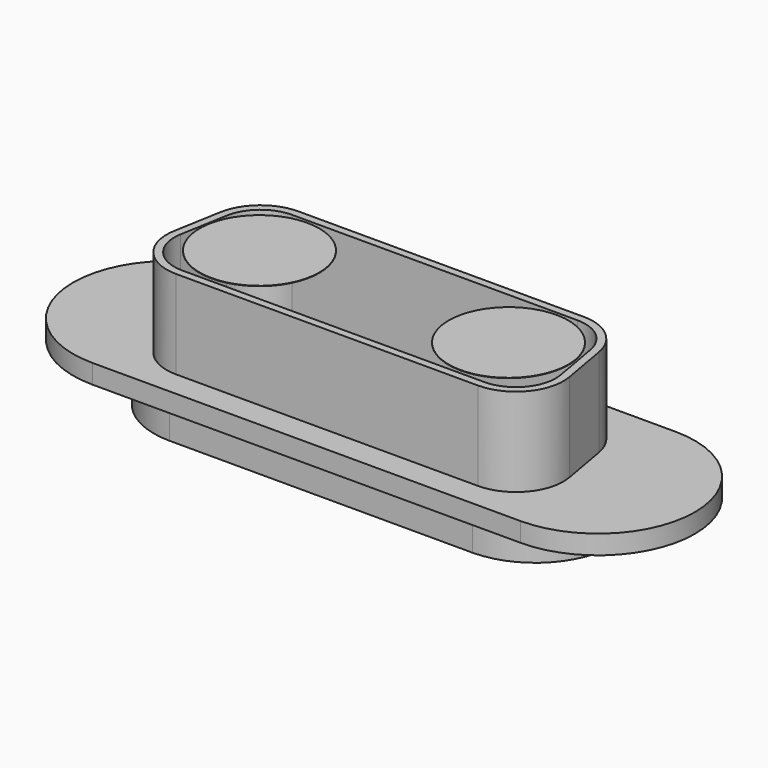
from build123d import *

# Parameters (mm, degrees)
F1_DEPTH      = 1.27
F3_DEPTH      = 2.413
F5_DEPTH      = 3.0988
F6_DEPTH      = 0.254
F8_DEPTH      = 3.684
F8_DEPTH_BACK = 5.8674
F9_DEPTH      = 5.8674
F11_DEPTH     = 0.0254


# Not quite as in the source:
# - an extrude ends at something that could not be found from the text; its depth is read off the source's solid


with BuildPart() as f1:
    # F0 (on Top) → F1 (new body)
    with BuildSketch(Plane.XY):
        with BuildLine():
            ThreePointArc((-14.2113, 6.4262), (-20.6375, 0), (-14.2113, -6.4262))
            Line((-14.2113, -6.4262), (14.2113, -6.4262))
            ThreePointArc((14.2113, -6.4262), (20.6375, 0), (14.2113, 6.4262))
            Line((14.2113, 6.4262), (-14.2113, 6.4262))
        make_face()
    extrude(amount=F1_DEPTH)

    # F2 (on face) → F3 (join)
    with BuildSketch(Plane(origin=(0, 0, 0), x_dir=(1, 0, 0), z_dir=(0, 0, -1))):
        with BuildLine():
            ThreePointArc((-10.0457, 5.2324), (-15.2781, 0), (-10.0457, -5.2324))
            Line((-10.0457, -5.2324), (10.0457, -5.2324))
            ThreePointArc((10.0457, -5.2324), (15.2781, 0), (10.0457, 5.2324))
            Line((10.0457, 5.2324), (-10.0457, 5.2324))
        make_face()
    extrude(amount=F3_DEPTH)

    # F4 (on face) → F5 (cut)
    with BuildSketch(Plane(origin=(0, 0, -2.413), x_dir=(1, 0, 0), z_dir=(0, 0, -1))):
        with BuildLine():
            ThreePointArc((10.0457, -4.3434), (14.3891, 0), (10.0457, 4.3434))
            Line((10.0457, 4.3434), (-10.0457, 4.3434))
            ThreePointArc((-10.0457, 4.3434), (-14.3891, 0), (-10.0457, -4.3434))
            Line((-10.0457, -4.3434), (10.0457, -4.3434))
        make_face()
    extrude(amount=-F5_DEPTH, mode=Mode.SUBTRACT)

    # F4 (on face) → F6 (cut)
    with BuildSketch(Plane(origin=(0, 0, -2.413), x_dir=(1, 0, 0), z_dir=(0, 0, -1))):
        with BuildLine():
            ThreePointArc((10.0457, -4.699), (14.7447, 0), (10.0457, 4.699))
            Line((10.0457, 4.699), (-10.0457, 4.699))
            ThreePointArc((-10.0457, 4.699), (-14.7447, 0), (-10.0457, -4.699))
            Line((-10.0457, -4.699), (10.0457, -4.699))
        make_face()
        with BuildLine():
            Line((-10.0457, 4.3434), (10.0457, 4.3434))
            ThreePointArc((10.0457, 4.3434), (14.3891, 0), (10.0457, -4.3434))
            Line((10.0457, -4.3434), (-10.0457, -4.3434))
            ThreePointArc((-10.0457, -4.3434), (-14.3891, 0), (-10.0457, 4.3434))
        make_face(mode=Mode.SUBTRACT)
    extrude(amount=-F6_DEPTH, mode=Mode.SUBTRACT)

    # F7 (on face) → F8 (cut, two sides)
    with BuildSketch(Plane.XY.offset(1.27)) as f8_sk:
        with BuildLine():
            Line((9.4649405416, 4.2164), (-9.4649405416, 4.2164))
            ThreePointArc((-9.4649405416, 4.2164), (-11.1629282913, 3.5983830009), (-12.0664087019, 2.0335090261))
            Line((-12.0664087019, 2.0335090261), (-12.6217681604, -1.1160909739))
            ThreePointArc((-12.6217681604, -1.1160909739), (-12.0438830009, -3.2727877497), (-10.0203, -4.2164))
            Line((-10.0203, -4.2164), (10.0203, -4.2164))
            ThreePointArc((10.0203, -4.2164), (12.0438830009, -3.2727877497), (12.6217681604, -1.1160909739))
            Line((12.6217681604, -1.1160909739), (12.0664087019, 2.0335090261))
            ThreePointArc((12.0664087019, 2.0335090261), (11.1629282913, 3.5983830009), (9.4649405416, 4.2164))
        make_face()
    extrude(amount=-F8_DEPTH, mode=Mode.SUBTRACT)
    extrude(f8_sk.sketch, amount=F8_DEPTH_BACK, mode=Mode.SUBTRACT)

    # F7 (on face) → F9 (join)
    with BuildSketch(Plane.XY.offset(1.27)):
        with BuildLine():
            Line((9.4649405416, 4.7244), (-9.4649405416, 4.7244))
            ThreePointArc((-9.4649405416, 4.7244), (-11.489464397, 3.987533578), (-12.5666910404, 2.1217223004))
            Line((-12.5666910404, 2.1217223004), (-13.1220504989, -1.0278776996))
            ThreePointArc((-13.1220504989, -1.0278776996), (-12.433033578, -3.5993238555), (-10.0203, -4.7244))
            Line((-10.0203, -4.7244), (10.0203, -4.7244))
            ThreePointArc((10.0203, -4.7244), (12.433033578, -3.5993238555), (13.1220504989, -1.0278776996))
            Line((13.1220504989, -1.0278776996), (12.5666910404, 2.1217223004))
            ThreePointArc((12.5666910404, 2.1217223004), (11.489464397, 3.987533578), (9.4649405416, 4.7244))
        make_face()
        with BuildLine():
            ThreePointArc((-12.0664087019, 2.0335090261), (-11.1629282913, 3.5983830009), (-9.4649405416, 4.2164))
            Line((-9.4649405416, 4.2164), (9.4649405416, 4.2164))
            ThreePointArc((9.4649405416, 4.2164), (11.1629282913, 3.5983830009), (12.0664087019, 2.0335090261))
            Line((12.0664087019, 2.0335090261), (12.6217681604, -1.1160909739))
            ThreePointArc((12.6217681604, -1.1160909739), (12.0438830009, -3.2727877497), (10.0203, -4.2164))
            Line((10.0203, -4.2164), (-10.0203, -4.2164))
            ThreePointArc((-10.0203, -4.2164), (-12.0438830009, -3.2727877497), (-12.6217681604, -1.1160909739))
            Line((-12.6217681604, -1.1160909739), (-12.0664087019, 2.0335090261))
        make_face(mode=Mode.SUBTRACT)
    extrude(amount=F9_DEPTH)


with BuildPart() as f11:
    # F10 (on face) → F11 (new body)
    with BuildSketch(Plane.XY.offset(7.1374)):
        with BuildLine():
            ThreePointArc((-4.2972876631, 0), (-7.9201383338, 3.9536477102), (-12.1744934415, 0.6891661563))
            ThreePointArc((-12.1744934415, 0.6891661563), (-8.6119369925, -3.9536477102), (-4.2972876631, 0))
        make_face()
    extrude(amount=F11_DEPTH)


with BuildPart() as f11b:
    # F10 (on face) → F11, piece 2 (new body)
    with BuildSketch(Plane.XY.offset(7.1374)):
        with BuildLine():
            ThreePointArc((12.2347876631, 0), (12.2196853686, 0.3458993835), (12.1744934226, 0.6891662634))
            ThreePointArc((12.1744934226, 0.6891662634), (4.3123899576, -0.3458993835), (12.2347876631, 0))
        make_face()
    extrude(amount=F11_DEPTH)


solid = Compound([f1.part, f11.part, f11b.part])
